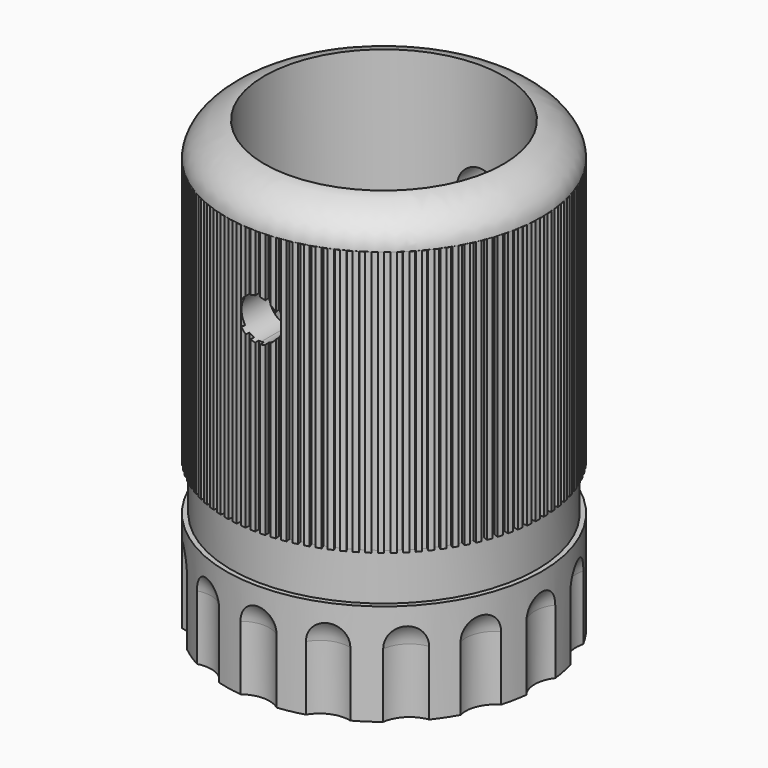
from build123d import *

# Parameters (mm, degrees)
F0_W      = 3.375
F0_H      = 14.874845035
F4_W      = 13.769172132
F4_H      = 12.0782218874
F5_DEPTH  = 25
F6_ANGLE  = 22.5
F7_ANGLE  = 45
F8_ANGLE  = 90
F9_ANGLE  = 180
F12_DEPTH = 22.5
F14_DEPTH = 26.8
F16_ANGLE = 3.6
F17_ANGLE = 7.2
F18_ANGLE = 14.4
F19_ANGLE = 28.8
F20_ANGLE = 57.6
F21_ANGLE = 115.2
F22_ANGLE = 57.6
F23_ANGLE = 57.6
F24_ANGLE = 14.4


# Not quite as in the source:
# - a feature names something its author has since deleted; it is built from what else it names


with BuildPart() as f1:
    # F0 (on Front) → F1 (revolve)
    with BuildSketch(Plane.XZ):
        with Locations((10.3625, -21.3657371884)):
            Rectangle(F0_W, F0_H)
        with BuildLine():
            add(Edge.make_bspline(
                [(12.05, 16.3568402941), (12.5508271158, 16.3568402941), (14.6515921131, 15.5552467799), (15.92, 13.8647258282), (15.92, 12.9073209008)],
                knots=[0, 0, 0, 0, 0.4828269764, 1, 1, 1, 1], degree=3))
            Line((12.05, 16.3568402941), (12.05, -13.9283146709))
            Line((12.05, -13.9283146709), (12.05, -28.8031597059))
            Line((12.05, -28.8031597059), (15.92, -28.8031597059))
            Line((15.92, -28.8031597059), (15.92, -18.5531597059))
            Line((15.92, -18.5531597059), (15.42, -18.5531597059))
            Line((15.42, -18.5531597059), (15.42, -13.8031597059))
            Line((15.42, -13.8031597059), (15.92, -13.8031597059))
            Line((15.92, -13.8031597059), (15.92, 12.2153926005))
            Line((15.92, 12.2153926005), (15.92, 12.9073209008))
        make_face()
    revolve(axis=Axis((0, 0, -6.2231597059), (0, 0, -1)))


with BuildPart() as f3:
    # F2 (on Front) → F3 (revolve)
    with BuildSketch(Plane.XZ):
        with BuildLine():
            Line((18.1992780417, -22.3115701228), (21.1992780417, -22.3115701228))
            ThreePointArc((21.1992780417, -22.3115701228), (20.3205983853, -20.1902497793), (18.1992780417, -19.3115701228))
            Line((18.1992780417, -19.3115701228), (18.1992780417, -22.3115701228))
        make_face()
        with BuildLine():
            ThreePointArc((18.1992780417, -25.3115701228), (20.3205983853, -24.4328904664), (21.1992780417, -22.3115701228))
            Line((21.1992780417, -22.3115701228), (18.1992780417, -22.3115701228))
            Line((18.1992780417, -22.3115701228), (18.1992780417, -25.3115701228))
        make_face()
        with BuildLine():
            Line((21.1992780417, -40.7387055457), (21.1992780417, -22.3115701228))
            ThreePointArc((21.1992780417, -22.3115701228), (20.3205983853, -24.4328904664), (18.1992780417, -25.3115701228))
            Line((18.1992780417, -25.3115701228), (18.1992780417, -40.7387055457))
            Line((18.1992780417, -40.7387055457), (21.1992780417, -40.7387055457))
        make_face()
    revolve(axis=Axis((18.1992780417, 0, -31.5251378343), (0, 0, -1)))


with BuildPart() as f5:
    # F4 (on Front) → F5 (new body)
    with BuildSketch(Plane.XZ):
        with Locations((-6.884586066, 37.2009221464)):
            Rectangle(F4_W, F4_H)
    extrude(amount=F5_DEPTH)


with BuildPart() as f6_1:
    # F6: copy of F3
    add(f3.part.rotate(Axis((0, 0, 37.2009221464), (0, 0, -1)), F6_ANGLE))


with BuildPart() as f7_1:
    # F7: copy of F6_1
    add(f6_1.part.rotate(Axis((0, 0, 37.2009221464), (0, 0, -1)), F7_ANGLE))


with BuildPart() as f7_2:
    # F7: copy of F3
    add(f3.part.rotate(Axis((0, 0, 37.2009221464), (0, 0, -1)), F7_ANGLE))


with BuildPart() as f8_1:
    # F8: copy of F3
    add(f3.part.rotate(Axis((0, 0, 37.2009221464), (0, 0, -1)), F8_ANGLE))


with BuildPart() as f8_2:
    # F8: copy of F6_1
    add(f6_1.part.rotate(Axis((0, 0, 37.2009221464), (0, 0, -1)), F8_ANGLE))


with BuildPart() as f8_3:
    # F8: copy of F7_2
    add(f7_2.part.rotate(Axis((0, 0, 37.2009221464), (0, 0, -1)), F8_ANGLE))


with BuildPart() as f8_4:
    # F8: copy of F7_1
    add(f7_1.part.rotate(Axis((0, 0, 37.2009221464), (0, 0, -1)), F8_ANGLE))


with BuildPart() as f9_1:
    # F9: copy of F3
    add(f3.part.rotate(Axis((0, 0, 37.2009221464), (0, 0, -1)), F9_ANGLE))


with BuildPart() as f9_2:
    # F9: copy of F6_1
    add(f6_1.part.rotate(Axis((0, 0, 37.2009221464), (0, 0, -1)), F9_ANGLE))


with BuildPart() as f9_3:
    # F9: copy of F7_2
    add(f7_2.part.rotate(Axis((0, 0, 37.2009221464), (0, 0, -1)), F9_ANGLE))


with BuildPart() as f9_4:
    # F9: copy of F7_1
    add(f7_1.part.rotate(Axis((0, 0, 37.2009221464), (0, 0, -1)), F9_ANGLE))


with BuildPart() as f9_5:
    # F9: copy of F8_1
    add(f8_1.part.rotate(Axis((0, 0, 37.2009221464), (0, 0, -1)), F9_ANGLE))


with BuildPart() as f9_6:
    # F9: copy of F8_2
    add(f8_2.part.rotate(Axis((0, 0, 37.2009221464), (0, 0, -1)), F9_ANGLE))


with BuildPart() as f9_7:
    # F9: copy of F8_3
    add(f8_3.part.rotate(Axis((0, 0, 37.2009221464), (0, 0, -1)), F9_ANGLE))


with BuildPart() as f9_8:
    # F9: copy of F8_4
    add(f8_4.part.rotate(Axis((0, 0, 37.2009221464), (0, 0, -1)), F9_ANGLE))


with BuildPart() as f1_1:
    add(f1.part)

    # F10: cut F8_4, F9_1, F9_2, F8_2, F8_3, F8_1, F7_1, F7_2, F6_1, F3, F9_8, F9_7, F9_6, F9_5, F9_4, F9_3
    add(f8_4.part, mode=Mode.SUBTRACT)
    add(f9_1.part, mode=Mode.SUBTRACT)
    add(f9_2.part, mode=Mode.SUBTRACT)
    add(f8_2.part, mode=Mode.SUBTRACT)
    add(f8_3.part, mode=Mode.SUBTRACT)
    add(f8_1.part, mode=Mode.SUBTRACT)
    add(f7_1.part, mode=Mode.SUBTRACT)
    add(f7_2.part, mode=Mode.SUBTRACT)
    add(f6_1.part, mode=Mode.SUBTRACT)
    add(f3.part, mode=Mode.SUBTRACT)
    add(f9_8.part, mode=Mode.SUBTRACT)
    add(f9_7.part, mode=Mode.SUBTRACT)
    add(f9_6.part, mode=Mode.SUBTRACT)
    add(f9_5.part, mode=Mode.SUBTRACT)
    add(f9_4.part, mode=Mode.SUBTRACT)
    add(f9_3.part, mode=Mode.SUBTRACT)

    # F11 (on Front) → F12 (cut, symmetric)
    with BuildSketch(Plane.XZ):
        with BuildLine():
            ThreePointArc((2.1105437549, 5.0743338652), (1.4923798011, 6.5667136663), (0, 7.1848776201))
            Line((0, 7.1848776201), (0, 2.9637901103))
            ThreePointArc((0, 2.9637901103), (1.4923798011, 3.5819540641), (2.1105437549, 5.0743338652))
        make_face()
        with BuildLine():
            Line((0, 2.9637901103), (0, 7.1848776201))
            ThreePointArc((0, 7.1848776201), (-2.1105437549, 5.0743338652), (0, 2.9637901103))
        make_face()
    extrude(amount=F12_DEPTH, both=True, mode=Mode.SUBTRACT)


with BuildPart() as f14:
    # F13 (on Top) → F14 (new body)
    with BuildSketch(Plane.XY):
        with BuildLine():
            ThreePointArc((-0.25, 15.7180119608), (0, 15.72), (0.25, 15.7180119608))
            Line((0.25, 15.7180119608), (0.25, 15.97))
            Line((0.25, 15.97), (-0.25, 15.97))
            Line((-0.25, 15.97), (-0.25, 15.7180119608))
        make_face()
        with BuildLine():
            Line((0.25, 15.47), (0.25, 15.7180119608))
            ThreePointArc((0.25, 15.7180119608), (0, 15.72), (-0.25, 15.7180119608))
            Line((-0.25, 15.7180119608), (-0.25, 15.47))
            Line((-0.25, 15.47), (0.25, 15.47))
        make_face()
    extrude(amount=F14_DEPTH)


with BuildPart() as f14_1:
    # F15: moved
    add(f14.part.moved(Location((0, 0, -13.9))))


with BuildPart() as f16_1:
    # F16: copy of F14
    add(f14_1.part.rotate(Axis((0, 0, 37.2009221464), (0, 0, -1)), F16_ANGLE))


with BuildPart() as f17_1:
    # F17: copy of F16_1
    add(f16_1.part.rotate(Axis((0, 0, 37.2009221464), (0, 0, -1)), F17_ANGLE))


with BuildPart() as f17_2:
    # F17: copy of F14
    add(f14_1.part.rotate(Axis((0, 0, 37.2009221464), (0, 0, -1)), F17_ANGLE))


with BuildPart() as f18_1:
    # F18: copy of F17_1
    add(f17_1.part.rotate(Axis((0, 0, 37.2009221464), (0, 0, -1)), F18_ANGLE))


with BuildPart() as f18_2:
    # F18: copy of F17_2
    add(f17_2.part.rotate(Axis((0, 0, 37.2009221464), (0, 0, -1)), F18_ANGLE))


with BuildPart() as f18_3:
    # F18: copy of F16_1
    add(f16_1.part.rotate(Axis((0, 0, 37.2009221464), (0, 0, -1)), F18_ANGLE))


with BuildPart() as f18_4:
    # F18: copy of F14
    add(f14_1.part.rotate(Axis((0, 0, 37.2009221464), (0, 0, -1)), F18_ANGLE))


with BuildPart() as f19_1:
    # F19: copy of F18_1
    add(f18_1.part.rotate(Axis((0, 0, 37.2009221464), (0, 0, -1)), F19_ANGLE))


with BuildPart() as f19_2:
    # F19: copy of F18_2
    add(f18_2.part.rotate(Axis((0, 0, 37.2009221464), (0, 0, -1)), F19_ANGLE))


with BuildPart() as f19_3:
    # F19: copy of F18_3
    add(f18_3.part.rotate(Axis((0, 0, 37.2009221464), (0, 0, -1)), F19_ANGLE))


with BuildPart() as f19_4:
    # F19: copy of F18_4
    add(f18_4.part.rotate(Axis((0, 0, 37.2009221464), (0, 0, -1)), F19_ANGLE))


with BuildPart() as f19_5:
    # F19: copy of F17_1
    add(f17_1.part.rotate(Axis((0, 0, 37.2009221464), (0, 0, -1)), F19_ANGLE))


with BuildPart() as f19_6:
    # F19: copy of F17_2
    add(f17_2.part.rotate(Axis((0, 0, 37.2009221464), (0, 0, -1)), F19_ANGLE))


with BuildPart() as f19_7:
    # F19: copy of F16_1
    add(f16_1.part.rotate(Axis((0, 0, 37.2009221464), (0, 0, -1)), F19_ANGLE))


with BuildPart() as f19_8:
    # F19: copy of F14
    add(f14_1.part.rotate(Axis((0, 0, 37.2009221464), (0, 0, -1)), F19_ANGLE))


with BuildPart() as f20_1:
    # F20: copy of F14
    add(f14_1.part.rotate(Axis((0, 0, 37.2009221464), (0, 0, -1)), F20_ANGLE))


with BuildPart() as f20_2:
    # F20: copy of F16_1
    add(f16_1.part.rotate(Axis((0, 0, 37.2009221464), (0, 0, -1)), F20_ANGLE))


with BuildPart() as f20_3:
    # F20: copy of F17_2
    add(f17_2.part.rotate(Axis((0, 0, 37.2009221464), (0, 0, -1)), F20_ANGLE))


with BuildPart() as f20_4:
    # F20: copy of F17_1
    add(f17_1.part.rotate(Axis((0, 0, 37.2009221464), (0, 0, -1)), F20_ANGLE))


with BuildPart() as f20_5:
    # F20: copy of F18_4
    add(f18_4.part.rotate(Axis((0, 0, 37.2009221464), (0, 0, -1)), F20_ANGLE))


with BuildPart() as f20_6:
    # F20: copy of F18_3
    add(f18_3.part.rotate(Axis((0, 0, 37.2009221464), (0, 0, -1)), F20_ANGLE))


with BuildPart() as f20_7:
    # F20: copy of F18_2
    add(f18_2.part.rotate(Axis((0, 0, 37.2009221464), (0, 0, -1)), F20_ANGLE))


with BuildPart() as f20_8:
    # F20: copy of F18_1
    add(f18_1.part.rotate(Axis((0, 0, 37.2009221464), (0, 0, -1)), F20_ANGLE))


with BuildPart() as f20_9:
    # F20: copy of F19_8
    add(f19_8.part.rotate(Axis((0, 0, 37.2009221464), (0, 0, -1)), F20_ANGLE))


with BuildPart() as f20_10:
    # F20: copy of F19_7
    add(f19_7.part.rotate(Axis((0, 0, 37.2009221464), (0, 0, -1)), F20_ANGLE))


with BuildPart() as f20_11:
    # F20: copy of F19_6
    add(f19_6.part.rotate(Axis((0, 0, 37.2009221464), (0, 0, -1)), F20_ANGLE))


with BuildPart() as f20_12:
    # F20: copy of F19_5
    add(f19_5.part.rotate(Axis((0, 0, 37.2009221464), (0, 0, -1)), F20_ANGLE))


with BuildPart() as f20_13:
    # F20: copy of F19_4
    add(f19_4.part.rotate(Axis((0, 0, 37.2009221464), (0, 0, -1)), F20_ANGLE))


with BuildPart() as f20_14:
    # F20: copy of F19_3
    add(f19_3.part.rotate(Axis((0, 0, 37.2009221464), (0, 0, -1)), F20_ANGLE))


with BuildPart() as f20_15:
    # F20: copy of F19_2
    add(f19_2.part.rotate(Axis((0, 0, 37.2009221464), (0, 0, -1)), F20_ANGLE))


with BuildPart() as f20_16:
    # F20: copy of F19_1
    add(f19_1.part.rotate(Axis((0, 0, 37.2009221464), (0, 0, -1)), F20_ANGLE))


with BuildPart() as f21_1:
    # F21: copy of F14
    add(f14_1.part.rotate(Axis((0, 0, 37.2009221464), (0, 0, -1)), F21_ANGLE))


with BuildPart() as f21_2:
    # F21: copy of F16_1
    add(f16_1.part.rotate(Axis((0, 0, 37.2009221464), (0, 0, -1)), F21_ANGLE))


with BuildPart() as f21_3:
    # F21: copy of F17_2
    add(f17_2.part.rotate(Axis((0, 0, 37.2009221464), (0, 0, -1)), F21_ANGLE))


with BuildPart() as f21_4:
    # F21: copy of F17_1
    add(f17_1.part.rotate(Axis((0, 0, 37.2009221464), (0, 0, -1)), F21_ANGLE))


with BuildPart() as f21_5:
    # F21: copy of F18_4
    add(f18_4.part.rotate(Axis((0, 0, 37.2009221464), (0, 0, -1)), F21_ANGLE))


with BuildPart() as f21_6:
    # F21: copy of F18_3
    add(f18_3.part.rotate(Axis((0, 0, 37.2009221464), (0, 0, -1)), F21_ANGLE))


with BuildPart() as f21_7:
    # F21: copy of F18_2
    add(f18_2.part.rotate(Axis((0, 0, 37.2009221464), (0, 0, -1)), F21_ANGLE))


with BuildPart() as f21_8:
    # F21: copy of F18_1
    add(f18_1.part.rotate(Axis((0, 0, 37.2009221464), (0, 0, -1)), F21_ANGLE))


with BuildPart() as f21_9:
    # F21: copy of F19_8
    add(f19_8.part.rotate(Axis((0, 0, 37.2009221464), (0, 0, -1)), F21_ANGLE))


with BuildPart() as f21_10:
    # F21: copy of F19_7
    add(f19_7.part.rotate(Axis((0, 0, 37.2009221464), (0, 0, -1)), F21_ANGLE))


with BuildPart() as f21_11:
    # F21: copy of F19_6
    add(f19_6.part.rotate(Axis((0, 0, 37.2009221464), (0, 0, -1)), F21_ANGLE))


with BuildPart() as f21_12:
    # F21: copy of F19_5
    add(f19_5.part.rotate(Axis((0, 0, 37.2009221464), (0, 0, -1)), F21_ANGLE))


with BuildPart() as f21_13:
    # F21: copy of F19_4
    add(f19_4.part.rotate(Axis((0, 0, 37.2009221464), (0, 0, -1)), F21_ANGLE))


with BuildPart() as f21_14:
    # F21: copy of F19_3
    add(f19_3.part.rotate(Axis((0, 0, 37.2009221464), (0, 0, -1)), F21_ANGLE))


with BuildPart() as f21_15:
    # F21: copy of F19_2
    add(f19_2.part.rotate(Axis((0, 0, 37.2009221464), (0, 0, -1)), F21_ANGLE))


with BuildPart() as f21_16:
    # F21: copy of F19_1
    add(f19_1.part.rotate(Axis((0, 0, 37.2009221464), (0, 0, -1)), F21_ANGLE))


with BuildPart() as f21_17:
    # F21: copy of F20_1
    add(f20_1.part.rotate(Axis((0, 0, 37.2009221464), (0, 0, -1)), F21_ANGLE))


with BuildPart() as f21_18:
    # F21: copy of F20_2
    add(f20_2.part.rotate(Axis((0, 0, 37.2009221464), (0, 0, -1)), F21_ANGLE))


with BuildPart() as f21_19:
    # F21: copy of F20_3
    add(f20_3.part.rotate(Axis((0, 0, 37.2009221464), (0, 0, -1)), F21_ANGLE))


with BuildPart() as f21_20:
    # F21: copy of F20_4
    add(f20_4.part.rotate(Axis((0, 0, 37.2009221464), (0, 0, -1)), F21_ANGLE))


with BuildPart() as f21_21:
    # F21: copy of F20_5
    add(f20_5.part.rotate(Axis((0, 0, 37.2009221464), (0, 0, -1)), F21_ANGLE))


with BuildPart() as f21_22:
    # F21: copy of F20_6
    add(f20_6.part.rotate(Axis((0, 0, 37.2009221464), (0, 0, -1)), F21_ANGLE))


with BuildPart() as f21_23:
    # F21: copy of F20_7
    add(f20_7.part.rotate(Axis((0, 0, 37.2009221464), (0, 0, -1)), F21_ANGLE))


with BuildPart() as f21_24:
    # F21: copy of F20_8
    add(f20_8.part.rotate(Axis((0, 0, 37.2009221464), (0, 0, -1)), F21_ANGLE))


with BuildPart() as f21_25:
    # F21: copy of F20_9
    add(f20_9.part.rotate(Axis((0, 0, 37.2009221464), (0, 0, -1)), F21_ANGLE))


with BuildPart() as f21_26:
    # F21: copy of F20_10
    add(f20_10.part.rotate(Axis((0, 0, 37.2009221464), (0, 0, -1)), F21_ANGLE))


with BuildPart() as f21_27:
    # F21: copy of F20_11
    add(f20_11.part.rotate(Axis((0, 0, 37.2009221464), (0, 0, -1)), F21_ANGLE))


with BuildPart() as f21_28:
    # F21: copy of F20_12
    add(f20_12.part.rotate(Axis((0, 0, 37.2009221464), (0, 0, -1)), F21_ANGLE))


with BuildPart() as f21_29:
    # F21: copy of F20_13
    add(f20_13.part.rotate(Axis((0, 0, 37.2009221464), (0, 0, -1)), F21_ANGLE))


with BuildPart() as f21_30:
    # F21: copy of F20_14
    add(f20_14.part.rotate(Axis((0, 0, 37.2009221464), (0, 0, -1)), F21_ANGLE))


with BuildPart() as f21_31:
    # F21: copy of F20_15
    add(f20_15.part.rotate(Axis((0, 0, 37.2009221464), (0, 0, -1)), F21_ANGLE))


with BuildPart() as f21_32:
    # F21: copy of F20_16
    add(f20_16.part.rotate(Axis((0, 0, 37.2009221464), (0, 0, -1)), F21_ANGLE))


with BuildPart() as f22_1:
    # F22: copy of F21_32
    add(f21_32.part.rotate(Axis((0, 0, 37.2009221464), (0, 0, -1)), F22_ANGLE))


with BuildPart() as f22_2:
    # F22: copy of F21_31
    add(f21_31.part.rotate(Axis((0, 0, 37.2009221464), (0, 0, -1)), F22_ANGLE))


with BuildPart() as f22_3:
    # F22: copy of F21_30
    add(f21_30.part.rotate(Axis((0, 0, 37.2009221464), (0, 0, -1)), F22_ANGLE))


with BuildPart() as f22_4:
    # F22: copy of F21_29
    add(f21_29.part.rotate(Axis((0, 0, 37.2009221464), (0, 0, -1)), F22_ANGLE))


with BuildPart() as f22_5:
    # F22: copy of F21_28
    add(f21_28.part.rotate(Axis((0, 0, 37.2009221464), (0, 0, -1)), F22_ANGLE))


with BuildPart() as f22_6:
    # F22: copy of F21_27
    add(f21_27.part.rotate(Axis((0, 0, 37.2009221464), (0, 0, -1)), F22_ANGLE))


with BuildPart() as f22_7:
    # F22: copy of F21_26
    add(f21_26.part.rotate(Axis((0, 0, 37.2009221464), (0, 0, -1)), F22_ANGLE))


with BuildPart() as f22_8:
    # F22: copy of F21_25
    add(f21_25.part.rotate(Axis((0, 0, 37.2009221464), (0, 0, -1)), F22_ANGLE))


with BuildPart() as f22_9:
    # F22: copy of F21_24
    add(f21_24.part.rotate(Axis((0, 0, 37.2009221464), (0, 0, -1)), F22_ANGLE))


with BuildPart() as f22_10:
    # F22: copy of F21_23
    add(f21_23.part.rotate(Axis((0, 0, 37.2009221464), (0, 0, -1)), F22_ANGLE))


with BuildPart() as f22_11:
    # F22: copy of F21_22
    add(f21_22.part.rotate(Axis((0, 0, 37.2009221464), (0, 0, -1)), F22_ANGLE))


with BuildPart() as f22_12:
    # F22: copy of F21_21
    add(f21_21.part.rotate(Axis((0, 0, 37.2009221464), (0, 0, -1)), F22_ANGLE))


with BuildPart() as f22_13:
    # F22: copy of F21_20
    add(f21_20.part.rotate(Axis((0, 0, 37.2009221464), (0, 0, -1)), F22_ANGLE))


with BuildPart() as f22_14:
    # F22: copy of F21_19
    add(f21_19.part.rotate(Axis((0, 0, 37.2009221464), (0, 0, -1)), F22_ANGLE))


with BuildPart() as f22_15:
    # F22: copy of F21_18
    add(f21_18.part.rotate(Axis((0, 0, 37.2009221464), (0, 0, -1)), F22_ANGLE))


with BuildPart() as f22_16:
    # F22: copy of F21_17
    add(f21_17.part.rotate(Axis((0, 0, 37.2009221464), (0, 0, -1)), F22_ANGLE))


with BuildPart() as f23_1:
    # F23: copy of F22_1
    add(f22_1.part.rotate(Axis((0, 0, 37.2009221464), (0, 0, -1)), F23_ANGLE))


with BuildPart() as f23_2:
    # F23: copy of F22_2
    add(f22_2.part.rotate(Axis((0, 0, 37.2009221464), (0, 0, -1)), F23_ANGLE))


with BuildPart() as f23_3:
    # F23: copy of F22_3
    add(f22_3.part.rotate(Axis((0, 0, 37.2009221464), (0, 0, -1)), F23_ANGLE))


with BuildPart() as f23_4:
    # F23: copy of F22_4
    add(f22_4.part.rotate(Axis((0, 0, 37.2009221464), (0, 0, -1)), F23_ANGLE))


with BuildPart() as f23_5:
    # F23: copy of F22_5
    add(f22_5.part.rotate(Axis((0, 0, 37.2009221464), (0, 0, -1)), F23_ANGLE))


with BuildPart() as f23_6:
    # F23: copy of F22_6
    add(f22_6.part.rotate(Axis((0, 0, 37.2009221464), (0, 0, -1)), F23_ANGLE))


with BuildPart() as f23_7:
    # F23: copy of F22_7
    add(f22_7.part.rotate(Axis((0, 0, 37.2009221464), (0, 0, -1)), F23_ANGLE))


with BuildPart() as f23_8:
    # F23: copy of F22_8
    add(f22_8.part.rotate(Axis((0, 0, 37.2009221464), (0, 0, -1)), F23_ANGLE))


with BuildPart() as f23_9:
    # F23: copy of F22_9
    add(f22_9.part.rotate(Axis((0, 0, 37.2009221464), (0, 0, -1)), F23_ANGLE))


with BuildPart() as f23_10:
    # F23: copy of F22_10
    add(f22_10.part.rotate(Axis((0, 0, 37.2009221464), (0, 0, -1)), F23_ANGLE))


with BuildPart() as f23_11:
    # F23: copy of F22_11
    add(f22_11.part.rotate(Axis((0, 0, 37.2009221464), (0, 0, -1)), F23_ANGLE))


with BuildPart() as f23_12:
    # F23: copy of F22_12
    add(f22_12.part.rotate(Axis((0, 0, 37.2009221464), (0, 0, -1)), F23_ANGLE))


with BuildPart() as f23_13:
    # F23: copy of F22_13
    add(f22_13.part.rotate(Axis((0, 0, 37.2009221464), (0, 0, -1)), F23_ANGLE))


with BuildPart() as f23_14:
    # F23: copy of F22_14
    add(f22_14.part.rotate(Axis((0, 0, 37.2009221464), (0, 0, -1)), F23_ANGLE))


with BuildPart() as f23_15:
    # F23: copy of F22_15
    add(f22_15.part.rotate(Axis((0, 0, 37.2009221464), (0, 0, -1)), F23_ANGLE))


with BuildPart() as f23_16:
    # F23: copy of F22_16
    add(f22_16.part.rotate(Axis((0, 0, 37.2009221464), (0, 0, -1)), F23_ANGLE))


with BuildPart() as f24_1:
    # F24: copy of F23_1
    add(f23_1.part.rotate(Axis((0, 0, 37.2009221464), (0, 0, -1)), F24_ANGLE))


with BuildPart() as f24_2:
    # F24: copy of F23_2
    add(f23_2.part.rotate(Axis((0, 0, 37.2009221464), (0, 0, -1)), F24_ANGLE))


with BuildPart() as f24_3:
    # F24: copy of F23_3
    add(f23_3.part.rotate(Axis((0, 0, 37.2009221464), (0, 0, -1)), F24_ANGLE))


with BuildPart() as f24_4:
    # F24: copy of F23_4
    add(f23_4.part.rotate(Axis((0, 0, 37.2009221464), (0, 0, -1)), F24_ANGLE))


with BuildPart() as f1_2:
    add(f1_1.part)

    # F25: cut F23_12, F19_3, F23_9, F23_4, F23_13, F23_10, F23_2, F21_4, F23_14, F23_6, F22_7, F23_7, F19_1, F19_4, F18_2, F18_1, F23_8, F23_3, F20_11, F19_6, F20_14, F20_8, F22_10, F20_16, F21_7, F23_11, F22_2, F24_2, F22_12, F20_10, F22_4, F23_5, F22_14, F22_6, F19_7, F21_1, F20_2, F20_3, F22_16, F21_2, F23_15, F21_3, F21_17, F23_16, F22_15, F22_9, F22_1, F21_9, F21_5, F20_4, F21_13, F20_13, F19_5, F20_9, F20_6, F19_2, F20_15, F17_2, F17_1, F18_4, F18_3, F19_8, F20_1, F22_3, F21_31, F21_25, F21_15, F22_11, F21_32, F21_10, F21_18, F22_8, F21_12, F21_19, F21_14, F21_30, F20_7, F20_12, F21_11, F21_8, F21_22, F21_27, F24_4, F20_5, F21_6, F21_16, F21_20, F23_1, F21_21, F21_28, F22_13, F21_29, F24_3, F21_26, F21_24, F22_5, F16_1, F14, F24_1, F21_23
    add(f23_12.part, mode=Mode.SUBTRACT)
    add(f19_3.part, mode=Mode.SUBTRACT)
    add(f23_9.part, mode=Mode.SUBTRACT)
    add(f23_4.part, mode=Mode.SUBTRACT)
    add(f23_13.part, mode=Mode.SUBTRACT)
    add(f23_10.part, mode=Mode.SUBTRACT)
    add(f23_2.part, mode=Mode.SUBTRACT)
    add(f21_4.part, mode=Mode.SUBTRACT)
    add(f23_14.part, mode=Mode.SUBTRACT)
    add(f23_6.part, mode=Mode.SUBTRACT)
    add(f22_7.part, mode=Mode.SUBTRACT)
    add(f23_7.part, mode=Mode.SUBTRACT)
    add(f19_1.part, mode=Mode.SUBTRACT)
    add(f19_4.part, mode=Mode.SUBTRACT)
    add(f18_2.part, mode=Mode.SUBTRACT)
    add(f18_1.part, mode=Mode.SUBTRACT)
    add(f23_8.part, mode=Mode.SUBTRACT)
    add(f23_3.part, mode=Mode.SUBTRACT)
    add(f20_11.part, mode=Mode.SUBTRACT)
    add(f19_6.part, mode=Mode.SUBTRACT)
    add(f20_14.part, mode=Mode.SUBTRACT)
    add(f20_8.part, mode=Mode.SUBTRACT)
    add(f22_10.part, mode=Mode.SUBTRACT)
    add(f20_16.part, mode=Mode.SUBTRACT)
    add(f21_7.part, mode=Mode.SUBTRACT)
    add(f23_11.part, mode=Mode.SUBTRACT)
    add(f22_2.part, mode=Mode.SUBTRACT)
    add(f24_2.part, mode=Mode.SUBTRACT)
    add(f22_12.part, mode=Mode.SUBTRACT)
    add(f20_10.part, mode=Mode.SUBTRACT)
    add(f22_4.part, mode=Mode.SUBTRACT)
    add(f23_5.part, mode=Mode.SUBTRACT)
    add(f22_14.part, mode=Mode.SUBTRACT)
    add(f22_6.part, mode=Mode.SUBTRACT)
    add(f19_7.part, mode=Mode.SUBTRACT)
    add(f21_1.part, mode=Mode.SUBTRACT)
    add(f20_2.part, mode=Mode.SUBTRACT)
    add(f20_3.part, mode=Mode.SUBTRACT)
    add(f22_16.part, mode=Mode.SUBTRACT)
    add(f21_2.part, mode=Mode.SUBTRACT)
    add(f23_15.part, mode=Mode.SUBTRACT)
    add(f21_3.part, mode=Mode.SUBTRACT)
    add(f21_17.part, mode=Mode.SUBTRACT)
    add(f23_16.part, mode=Mode.SUBTRACT)
    add(f22_15.part, mode=Mode.SUBTRACT)
    add(f22_9.part, mode=Mode.SUBTRACT)
    add(f22_1.part, mode=Mode.SUBTRACT)
    add(f21_9.part, mode=Mode.SUBTRACT)
    add(f21_5.part, mode=Mode.SUBTRACT)
    add(f20_4.part, mode=Mode.SUBTRACT)
    add(f21_13.part, mode=Mode.SUBTRACT)
    add(f20_13.part, mode=Mode.SUBTRACT)
    add(f19_5.part, mode=Mode.SUBTRACT)
    add(f20_9.part, mode=Mode.SUBTRACT)
    add(f20_6.part, mode=Mode.SUBTRACT)
    add(f19_2.part, mode=Mode.SUBTRACT)
    add(f20_15.part, mode=Mode.SUBTRACT)
    add(f17_2.part, mode=Mode.SUBTRACT)
    add(f17_1.part, mode=Mode.SUBTRACT)
    add(f18_4.part, mode=Mode.SUBTRACT)
    add(f18_3.part, mode=Mode.SUBTRACT)
    add(f19_8.part, mode=Mode.SUBTRACT)
    add(f20_1.part, mode=Mode.SUBTRACT)
    add(f22_3.part, mode=Mode.SUBTRACT)
    add(f21_31.part, mode=Mode.SUBTRACT)
    add(f21_25.part, mode=Mode.SUBTRACT)
    add(f21_15.part, mode=Mode.SUBTRACT)
    add(f22_11.part, mode=Mode.SUBTRACT)
    add(f21_32.part, mode=Mode.SUBTRACT)
    add(f21_10.part, mode=Mode.SUBTRACT)
    add(f21_18.part, mode=Mode.SUBTRACT)
    add(f22_8.part, mode=Mode.SUBTRACT)
    add(f21_12.part, mode=Mode.SUBTRACT)
    add(f21_19.part, mode=Mode.SUBTRACT)
    add(f21_14.part, mode=Mode.SUBTRACT)
    add(f21_30.part, mode=Mode.SUBTRACT)
    add(f20_7.part, mode=Mode.SUBTRACT)
    add(f20_12.part, mode=Mode.SUBTRACT)
    add(f21_11.part, mode=Mode.SUBTRACT)
    add(f21_8.part, mode=Mode.SUBTRACT)
    add(f21_22.part, mode=Mode.SUBTRACT)
    add(f21_27.part, mode=Mode.SUBTRACT)
    add(f24_4.part, mode=Mode.SUBTRACT)
    add(f20_5.part, mode=Mode.SUBTRACT)
    add(f21_6.part, mode=Mode.SUBTRACT)
    add(f21_16.part, mode=Mode.SUBTRACT)
    add(f21_20.part, mode=Mode.SUBTRACT)
    add(f23_1.part, mode=Mode.SUBTRACT)
    add(f21_21.part, mode=Mode.SUBTRACT)
    add(f21_28.part, mode=Mode.SUBTRACT)
    add(f22_13.part, mode=Mode.SUBTRACT)
    add(f21_29.part, mode=Mode.SUBTRACT)
    add(f24_3.part, mode=Mode.SUBTRACT)
    add(f21_26.part, mode=Mode.SUBTRACT)
    add(f21_24.part, mode=Mode.SUBTRACT)
    add(f22_5.part, mode=Mode.SUBTRACT)
    add(f16_1.part, mode=Mode.SUBTRACT)
    add(f14_1.part, mode=Mode.SUBTRACT)
    add(f24_1.part, mode=Mode.SUBTRACT)
    add(f21_23.part, mode=Mode.SUBTRACT)


solid = f1_2.part
